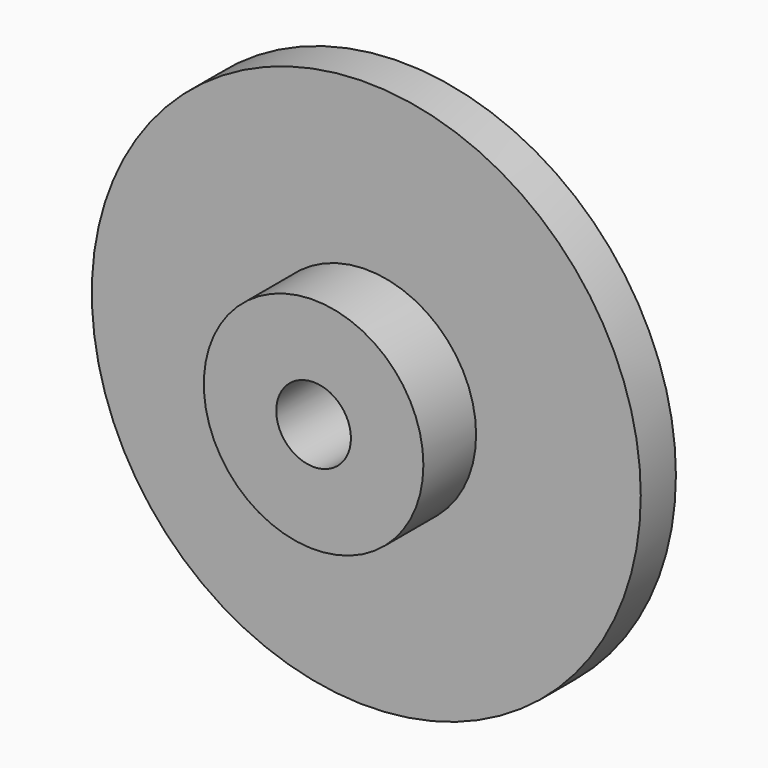
from build123d import *

# Parameters (mm, degrees)
F0_R          = 12.7
F1_DEPTH      = 12.7
F2_R          = 31.75
F3_DEPTH      = 5.08
F4_R          = 4.318
F5_DEPTH      = 12.701
F5_DEPTH_BACK = 95


# Not quite as in the source:
# - an extrude ends at something that could not be found from the text; its depth is read off the source's solid


with BuildPart() as f1:
    # F0 (on Front) → F1 (new body)
    with BuildSketch(Plane.XZ):
        Circle(F0_R)
    extrude(amount=F1_DEPTH)

    # F2 (on Front) → F3 (join)
    with BuildSketch(Plane.XZ):
        Circle(F2_R)
    extrude(amount=F3_DEPTH)

    # F4 (on Front) → F5 (cut, two sides)
    with BuildSketch(Plane.XZ) as f5_sk:
        Circle(F4_R)
    extrude(amount=F5_DEPTH, mode=Mode.SUBTRACT)
    extrude(f5_sk.sketch, amount=-F5_DEPTH_BACK, mode=Mode.SUBTRACT)


solid = f1.part
